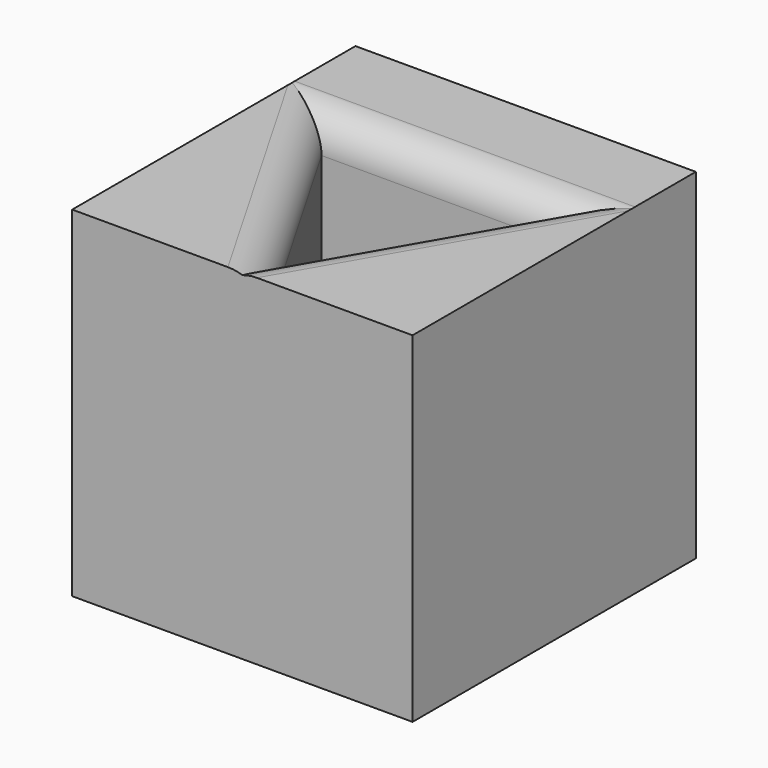
from build123d import *

# Parameters (mm, degrees)
F0_W         = 20
F0_H         = 20
F1_DEPTH     = 20.8070650697
F3_DEPTH     = 10
F4_T4_DEPTH  = 23.6433897602
F4_T10_DEPTH = 23.6433897602
F4_T15_DEPTH = 23.6433897602
F4_T20_DEPTH = 23.6433897602
F4_T26_DEPTH = 23.6433897602
F4_T32_DEPTH = 23.6433897602
F4_T39_DEPTH = 23.6433897602
F4_T44_DEPTH = 23.6433897602
F4_T52_DEPTH = 23.6433897602
F4_T57_DEPTH = 23.6433897602
F4_T65_DEPTH = 23.6433897602
F4_T70_DEPTH = 23.6433897602


# Not quite as in the source:
# - a fillet or chamfer that OpenCascade refuses, or shapes differently, is made with other operations: its cross-section is extruded or revolved along the edge and cut away or added


with BuildPart() as f1:
    # F0 (on Front) → F1 (new body)
    with BuildSketch(Plane.XZ):
        with Locations((10, 10)):
            Rectangle(F0_W, F0_H)
    extrude(amount=F1_DEPTH)

    # F2 (on face) → F3 (cut)
    with BuildSketch(Plane.XY.offset(20)):
        Polygon((10, -18.2805472855), (16.8216948801, -6.4650251595), (3.1783051199, -6.4650251595), align=None)
    extrude(amount=-F3_DEPTH, mode=Mode.SUBTRACT)

    # F4: fillet of radius 2 on 6 edges, made by hand


with BuildPart() as f4_tool2:
    # F4_s3 → F4_t4 (new body)
    with BuildSketch(Plane.YZ.offset(21.8216948801)):
        with BuildLine():
            ThreePointArc((-6.4650251595, 12), (-7.0508115971, 10.5857864376), (-8.4650251595, 10))
            Line((-8.4650251595, 10), (-6.4650251595, 10))
            Line((-6.4650251595, 10), (-6.4650251595, 12))
        make_face()
    extrude(amount=-F4_T4_DEPTH)

    split(bisect_by=Plane(origin=(-0.4157091722, -0.2400098025, 0), x_dir=(0, 0, 1), z_dir=(0.8660254038, 0.5, 0)), keep=Keep.TOP)

    split(bisect_by=Plane(origin=(15.4157091722, -8.9002638403, 0), x_dir=(0, 0, 1), z_dir=(-0.8660254038, 0.5, 0)), keep=Keep.TOP)


with BuildPart() as f1_1:
    add(f1.part)

    # F4_t1: union F4_tool2
    add(f4_tool2.part)


with BuildPart() as f4_tool8:
    # F4_s9 → F4_t10 (new body)
    with BuildSketch(Plane(origin=(-7.9157091722, -13.7104104641, 0), x_dir=(0, 0, 1), z_dir=(0.5, 0.8660254038, 0))):
        with BuildLine():
            ThreePointArc((12, 17.8005276806), (10.5857864376, 17.214741243), (10, 15.8005276806))
            Line((10, 15.8005276806), (10, 17.8005276806))
            Line((10, 17.8005276806), (12, 17.8005276806))
        make_face()
    extrude(amount=F4_T10_DEPTH)

    split(bisect_by=Plane(origin=(-0.4157091722, -0.2400098025, 0), x_dir=(0, 0, 1), z_dir=(0.8660254038, 0.5, 0)), keep=Keep.TOP)


with BuildPart() as f1_2:
    add(f1_1.part)

    # F4_t7: union F4_tool8
    add(f4_tool8.part)


with BuildPart() as f4_tool13:
    # F4_s14 → F4_t15 (new body)
    with BuildSketch(Plane(origin=(1.0940142921, -1.8948883381, 0), x_dir=(0, 0, 1), z_dir=(0.5, -0.8660254038, 0))):
        with BuildLine():
            ThreePointArc((12, 0.4800196049), (10.5857864376, -0.1057668327), (10, -1.5199803951))
            Line((10, -1.5199803951), (10, 0.4800196049))
            Line((10, 0.4800196049), (12, 0.4800196049))
        make_face()
    extrude(amount=F4_T15_DEPTH)

    split(bisect_by=Plane(origin=(15.4157091722, -8.9002638403, 0), x_dir=(0, 0, 1), z_dir=(-0.8660254038, 0.5, 0)), keep=Keep.TOP)


with BuildPart() as f1_3:
    add(f1_2.part)

    # F4_t12: union F4_tool13
    add(f4_tool13.part)


with BuildPart() as f4_tool18:
    # F4_s19 → F4_t20 (new body)
    with BuildSketch(Plane(origin=(-7.9157091722, -13.7104104641, 0), x_dir=(0, 0, 1), z_dir=(0.5, 0.8660254038, 0))):
        with BuildLine():
            ThreePointArc((20, 19.8005276806), (19.4142135624, 18.3863141182), (18, 17.8005276806))
            Line((18, 17.8005276806), (20, 17.8005276806))
            Line((20, 17.8005276806), (20, 19.8005276806))
        make_face()
    extrude(amount=F4_T20_DEPTH)

    split(bisect_by=Plane(origin=(-0.4157091722, -0.2400098025, 0), x_dir=(0, 0, 1), z_dir=(0.8660254038, 0.5, 0)), keep=Keep.TOP)

    split(bisect_by=Plane.XZ.offset(6.4650251595), keep=Keep.TOP)


with BuildPart() as f1_4:
    add(f1_3.part)

    # F4_t17: cut F4_tool18
    add(f4_tool18.part, mode=Mode.SUBTRACT)


with BuildPart() as f4_tool24:
    # F4_s25 → F4_t26 (new body)
    with BuildSketch(Plane(origin=(1.0940142921, -1.8948883381, 0), x_dir=(0, 0, 1), z_dir=(0.5, -0.8660254038, 0))):
        with BuildLine():
            ThreePointArc((20, 2.4800196049), (19.4142135624, 1.0658060425), (18, 0.4800196049))
            Line((18, 0.4800196049), (20, 0.4800196049))
            Line((20, 0.4800196049), (20, 2.4800196049))
        make_face()
    extrude(amount=F4_T26_DEPTH)

    split(bisect_by=Plane.XZ.offset(6.4650251595), keep=Keep.TOP)

    split(bisect_by=Plane(origin=(15.4157091722, -8.9002638403, 0), x_dir=(0, 0, 1), z_dir=(-0.8660254038, 0.5, 0)), keep=Keep.TOP)


with BuildPart() as f1_5:
    add(f1_4.part)

    # F4_t23: cut F4_tool24
    add(f4_tool24.part, mode=Mode.SUBTRACT)


with BuildPart() as f4_tool30:
    # F4_s31 → F4_t32 (new body)
    with BuildSketch(Plane.YZ.offset(21.8216948801)):
        with BuildLine():
            ThreePointArc((-4.4650251595, 20), (-5.8792387219, 19.4142135624), (-6.4650251595, 18))
            Line((-6.4650251595, 18), (-6.4650251595, 20))
            Line((-6.4650251595, 20), (-4.4650251595, 20))
        make_face()
    extrude(amount=-F4_T32_DEPTH)

    split(bisect_by=Plane(origin=(-0.4157091722, -0.2400098025, 0), x_dir=(0, 0, 1), z_dir=(0.8660254038, 0.5, 0)), keep=Keep.TOP)

    split(bisect_by=Plane(origin=(15.4157091722, -8.9002638403, 0), x_dir=(0, 0, 1), z_dir=(-0.8660254038, 0.5, 0)), keep=Keep.TOP)


with BuildPart() as f1_6:
    add(f1_5.part)

    # F4_t29: cut F4_tool30
    add(f4_tool30.part, mode=Mode.SUBTRACT)


with BuildPart() as f4_tool37:
    # F4_s38 → F4_t39 (new body)
    with BuildSketch(Plane(origin=(1.0940142921, -1.8948883381, 0), x_dir=(0, 0, 1), z_dir=(0.5, -0.8660254038, 0))):
        with BuildLine():
            ThreePointArc((20, 2.4800196049), (19.4142135624, 1.0658060425), (18, 0.4800196049))
            Line((18, 0.4800196049), (20, 0.4800196049))
            Line((20, 0.4800196049), (20, 2.4800196049))
        make_face()
    extrude(amount=F4_T39_DEPTH)

    split(bisect_by=Plane.XZ.offset(20.8070650697), keep=Keep.BOTTOM)

    split(bisect_by=Plane(origin=(15.4157091722, -8.9002638403, 0), x_dir=(0, 0, 1), z_dir=(0.8660254038, -0.5, 0)), keep=Keep.TOP)


with BuildPart() as f4_tool42:
    # F4_s43 → F4_t44 (new body)
    with BuildSketch(Plane(origin=(-7.9157091722, -13.7104104641, 0), x_dir=(0, 0, 1), z_dir=(0.5, 0.8660254038, 0))):
        with BuildLine():
            ThreePointArc((20, 19.8005276806), (19.4142135624, 18.3863141182), (18, 17.8005276806))
            Line((18, 17.8005276806), (20, 17.8005276806))
            Line((20, 17.8005276806), (20, 19.8005276806))
        make_face()
    extrude(amount=F4_T44_DEPTH)

    split(bisect_by=Plane.XZ.offset(20.8070650697), keep=Keep.BOTTOM)

    split(bisect_by=Plane(origin=(-0.4157091722, -0.2400098025, 0), x_dir=(0, 0, 1), z_dir=(-0.8660254038, -0.5, 0)), keep=Keep.TOP)


with BuildPart() as f4_tool37_1:
    add(f4_tool37.part)

    # F4_t47: intersect F4_tool42
    add(f4_tool42.part, mode=Mode.INTERSECT)


with BuildPart() as f1_7:
    add(f1_6.part)

    # F4_t35: cut F4_tool37
    add(f4_tool37_1.part, mode=Mode.SUBTRACT)


with BuildPart() as f4_tool50:
    # F4_s51 → F4_t52 (new body)
    with BuildSketch(Plane.YZ.offset(21.8216948801)):
        with BuildLine():
            ThreePointArc((-4.4650251595, 20), (-5.8792387219, 19.4142135624), (-6.4650251595, 18))
            Line((-6.4650251595, 18), (-6.4650251595, 20))
            Line((-6.4650251595, 20), (-4.4650251595, 20))
        make_face()
    extrude(amount=-F4_T52_DEPTH)

    split(bisect_by=Plane.YZ.offset(20), keep=Keep.BOTTOM)

    split(bisect_by=Plane(origin=(15.4157091722, -8.9002638403, 0), x_dir=(0, 0, 1), z_dir=(0.8660254038, -0.5, 0)), keep=Keep.TOP)


with BuildPart() as f4_tool55:
    # F4_s56 → F4_t57 (new body)
    with BuildSketch(Plane(origin=(-7.9157091722, -13.7104104641, 0), x_dir=(0, 0, 1), z_dir=(0.5, 0.8660254038, 0))):
        with BuildLine():
            ThreePointArc((20, 19.8005276806), (19.4142135624, 18.3863141182), (18, 17.8005276806))
            Line((18, 17.8005276806), (20, 17.8005276806))
            Line((20, 17.8005276806), (20, 19.8005276806))
        make_face()
    extrude(amount=F4_T57_DEPTH)

    split(bisect_by=Plane.YZ.offset(20), keep=Keep.BOTTOM)

    split(bisect_by=Plane.XZ.offset(6.4650251595), keep=Keep.BOTTOM)


with BuildPart() as f4_tool50_1:
    add(f4_tool50.part)

    # F4_t60: intersect F4_tool55
    add(f4_tool55.part, mode=Mode.INTERSECT)


with BuildPart() as f1_8:
    add(f1_7.part)

    # F4_t48: cut F4_tool50
    add(f4_tool50_1.part, mode=Mode.SUBTRACT)


with BuildPart() as f4_tool63:
    # F4_s64 → F4_t65 (new body)
    with BuildSketch(Plane(origin=(1.0940142921, -1.8948883381, 0), x_dir=(0, 0, 1), z_dir=(0.5, -0.8660254038, 0))):
        with BuildLine():
            ThreePointArc((20, 2.4800196049), (19.4142135624, 1.0658060425), (18, 0.4800196049))
            Line((18, 0.4800196049), (20, 0.4800196049))
            Line((20, 0.4800196049), (20, 2.4800196049))
        make_face()
    extrude(amount=F4_T65_DEPTH)

    split(bisect_by=Plane.YZ, keep=Keep.TOP)

    split(bisect_by=Plane.XZ.offset(6.4650251595), keep=Keep.BOTTOM)


with BuildPart() as f4_tool68:
    # F4_s69 → F4_t70 (new body)
    with BuildSketch(Plane.YZ.offset(21.8216948801)):
        with BuildLine():
            ThreePointArc((-4.4650251595, 20), (-5.8792387219, 19.4142135624), (-6.4650251595, 18))
            Line((-6.4650251595, 18), (-6.4650251595, 20))
            Line((-6.4650251595, 20), (-4.4650251595, 20))
        make_face()
    extrude(amount=-F4_T70_DEPTH)

    split(bisect_by=Plane.YZ, keep=Keep.TOP)

    split(bisect_by=Plane(origin=(-0.4157091722, -0.2400098025, 0), x_dir=(0, 0, 1), z_dir=(-0.8660254038, -0.5, 0)), keep=Keep.TOP)


with BuildPart() as f4_tool63_1:
    add(f4_tool63.part)

    # F4_t73: intersect F4_tool68
    add(f4_tool68.part, mode=Mode.INTERSECT)


with BuildPart() as f1_9:
    add(f1_8.part)

    # F4_t61: cut F4_tool63
    add(f4_tool63_1.part, mode=Mode.SUBTRACT)


solid = f1_9.part
